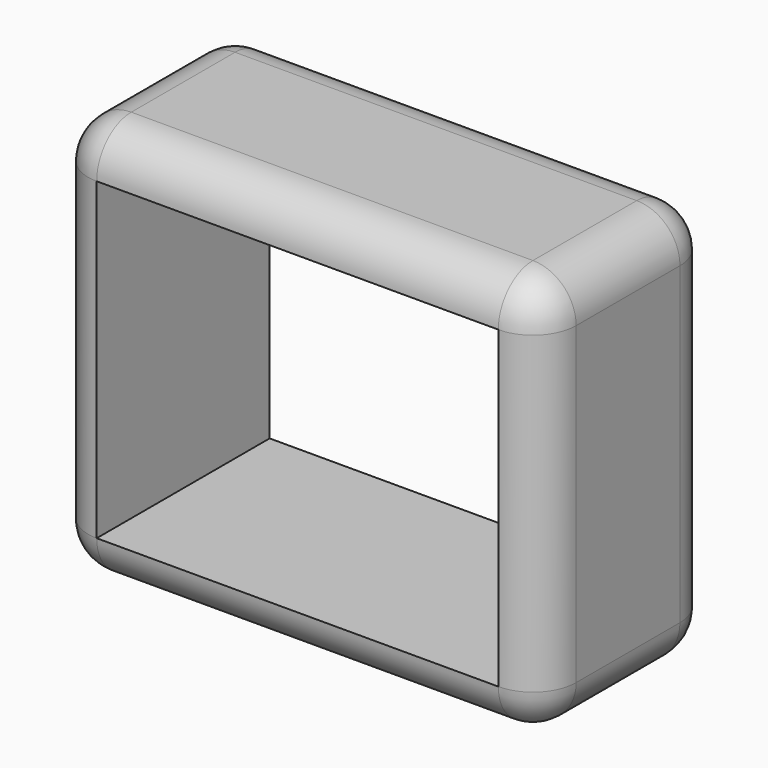
from build123d import *

# Parameters (mm, degrees)
F0_W         = 57.346759364
F0_H         = 47.0794383436
F1_DEPTH     = 25.4
F2_R         = 5.08
F3_T1_DEPTH  = 33.02
F3_T3_DEPTH  = 72.4794383436
F3_S7_W      = 5.08
F3_S7_H      = 5.08
F3_T8_DEPTH  = 5.08
F3_S13_W     = 5.08
F3_S13_H     = 5.08
F3_T14_DEPTH = 5.08
F4_T1_DEPTH  = 47.186759364
F4_T3_DEPTH  = 15.24
F4_T5_DEPTH  = 54.6994383436
F4_S9_W      = 5.08
F4_S9_H      = 5.08
F4_T10_DEPTH = 5.08
F4_S15_W     = 5.08
F4_S15_H     = 5.08
F4_T16_DEPTH = 5.08
F4_S21_W     = 5.08
F4_S21_H     = 5.08
F4_T22_DEPTH = 5.08
F5_T1_DEPTH  = 47.186759364
F5_T3_DEPTH  = 15.24
F5_S7_W      = 5.08
F5_S7_H      = 5.08
F5_T8_DEPTH  = 5.08
F5_S13_W     = 5.08
F5_S13_H     = 5.08
F5_T14_DEPTH = 5.08
F5_T18_ANGLE = 89.9999999979
F6_DEPTH     = 25.4


# Not quite as in the source:
# - a fillet or chamfer that OpenCascade refuses, or shapes differently, is made with other operations: its cross-section is extruded or revolved along the edge and cut away or added


with BuildPart() as f1:
    # F0 (on Front) → F1 (new body)
    with BuildSketch(Plane.XZ):
        with Locations((-1.5025353059, 0.5008457229)):
            Rectangle(F0_W, F0_H)
    extrude(amount=F1_DEPTH)

    # F2
    f2_edges = [f1.edges().sort_by_distance(p)[0] for p in [
        (-30.175915, -25.4, 0.500846),
        (-1.502535, -25.4, -23.038873),
        (27.170844, -25.4, 0.500846),
        (-1.502535, -25.4, 24.040565),
    ]]
    fillet(f2_edges, radius=F2_R)

    # F3: fillet of radius 5.08 on 3 edges, made by hand

    # F3_s2 → F3_t1 (cut)
    with BuildSketch(Plane.XZ.offset(-12.7)):
        with BuildLine():
            ThreePointArc((22.0908443761, 24.0405648947), (25.6829468245, 22.5526673431), (27.1708443761, 18.9605648947))
            Line((27.1708443761, 18.9605648947), (27.1708443761, 24.0405648947))
            Line((27.1708443761, 24.0405648947), (22.0908443761, 24.0405648947))
        make_face()
        with BuildLine():
            ThreePointArc((22.0908443761, -23.038873449), (25.6829468245, -21.5509758974), (27.1708443761, -17.958873449))
            Line((27.1708443761, -17.958873449), (27.1708443761, -23.038873449))
            Line((27.1708443761, -23.038873449), (22.0908443761, -23.038873449))
        make_face()
    extrude(amount=F3_T1_DEPTH, mode=Mode.SUBTRACT)

    # F3_s4 → F3_t3 (cut)
    with BuildSketch(Plane.XY.offset(-35.738873449)):
        with BuildLine():
            ThreePointArc((22.0908443761, 0), (25.6829468245, -1.4878975516), (27.1708443761, -5.08))
            Line((27.1708443761, -5.08), (27.1708443761, 0))
            Line((27.1708443761, 0), (22.0908443761, 0))
        make_face()
    extrude(amount=F3_T3_DEPTH, mode=Mode.SUBTRACT)


with BuildPart() as f3_tool6:
    # F3_s7 → F3_t8 (new body)
    with BuildSketch(Plane.XY.offset(-17.958873449)):
        with Locations((24.6308443761, -22.86)):
            Rectangle(F3_S7_W, F3_S7_H)
    extrude(amount=-F3_T8_DEPTH)

    # F3_s9 → F3_t10 (revolve, cut)
    with BuildSketch(Plane(origin=(22.0908443761, -20.32, -17.958873449), x_dir=(-0.7071067812, 0.7071067812, 0), z_dir=(-0.7071067812, -0.7071067812, 0))):
        with BuildLine():
            ThreePointArc((0, -5.08), (5.08, 0), (0, 5.08))
            Line((0, 5.08), (0, -5.08))
        make_face()
    revolve(axis=Axis((22.0908443761, -20.32, -17.958873449), (0, 0, -1)), mode=Mode.SUBTRACT)


with BuildPart() as f1_1:
    add(f1.part)

    # F3_t5: cut F3_tool6
    add(f3_tool6.part, mode=Mode.SUBTRACT)


with BuildPart() as f3_tool12:
    # F3_s13 → F3_t14 (new body)
    with BuildSketch(Plane.XY.offset(18.9605648947)):
        with Locations((24.6308443761, -22.86)):
            Rectangle(F3_S13_W, F3_S13_H)
    extrude(amount=F3_T14_DEPTH)

    # F3_s15 → F3_t16 (revolve, cut)
    with BuildSketch(Plane(origin=(22.0908443761, -20.32, 18.9605648947), x_dir=(-0.7071067812, 0.7071067812, 0), z_dir=(0.7071067812, 0.7071067812, 0))):
        with BuildLine():
            ThreePointArc((0, -5.08), (5.08, 0), (0, 5.08))
            Line((0, 5.08), (0, -5.08))
        make_face()
    revolve(axis=Axis((22.0908443761, -20.32, 18.9605648947), (0, 0, 1)), mode=Mode.SUBTRACT)


with BuildPart() as f1_2:
    add(f1_1.part)

    # F3_t11: cut F3_tool12
    add(f3_tool12.part, mode=Mode.SUBTRACT)

    # F4: fillet of radius 5.08 on 3 edges, made by hand

    # F4_s2 → F4_t1 (cut)
    with BuildSketch(Plane.YZ.offset(-25.0959149879)):
        with BuildLine():
            ThreePointArc((0, -17.958873449), (-1.4878975516, -21.5509758974), (-5.08, -23.038873449))
            Line((-5.08, -23.038873449), (0, -23.038873449))
            Line((0, -23.038873449), (0, -17.958873449))
        make_face()
    extrude(amount=F4_T1_DEPTH, mode=Mode.SUBTRACT)

    # F4_s4 → F4_t3 (cut)
    with BuildSketch(Plane.XZ.offset(5.08)):
        with BuildLine():
            ThreePointArc((-30.1759149879, -17.958873449), (-28.6880174363, -21.5509758974), (-25.0959149879, -23.038873449))
            Line((-25.0959149879, -23.038873449), (-30.1759149879, -23.038873449))
            Line((-30.1759149879, -23.038873449), (-30.1759149879, -17.958873449))
        make_face()
    extrude(amount=F4_T3_DEPTH, mode=Mode.SUBTRACT)

    # F4_s6 → F4_t5 (cut)
    with BuildSketch(Plane.XY.offset(-17.958873449)):
        with BuildLine():
            ThreePointArc((-30.1759149879, -5.08), (-28.6880174363, -1.4878975516), (-25.0959149879, 0))
            Line((-25.0959149879, 0), (-30.1759149879, 0))
            Line((-30.1759149879, 0), (-30.1759149879, -5.08))
        make_face()
    extrude(amount=F4_T5_DEPTH, mode=Mode.SUBTRACT)


with BuildPart() as f4_tool8:
    # F4_s9 → F4_t10 (new body)
    with BuildSketch(Plane.YZ.offset(-25.0959149879)):
        with Locations((-22.86, -20.498873449)):
            Rectangle(F4_S9_W, F4_S9_H)
    extrude(amount=-F4_T10_DEPTH)

    # F4_s11 → F4_t12 (revolve, cut)
    with BuildSketch(Plane(origin=(-25.0959149879, -20.32, -17.958873449), x_dir=(0, 0.7071067812, 0.7071067812), z_dir=(0, -0.7071067812, 0.7071067812))):
        with BuildLine():
            ThreePointArc((0, -5.08), (5.08, 0), (0, 5.08))
            Line((0, 5.08), (0, -5.08))
        make_face()
    revolve(axis=Axis((-25.0959149879, -20.32, -17.958873449), (-1, 0, 0)), mode=Mode.SUBTRACT)


with BuildPart() as f1_3:
    add(f1_2.part)

    # F4_t7: cut F4_tool8
    add(f4_tool8.part, mode=Mode.SUBTRACT)


with BuildPart() as f4_tool14:
    # F4_s15 → F4_t16 (new body)
    with BuildSketch(Plane.XZ.offset(5.08)):
        with Locations((24.6308443761, -20.498873449)):
            Rectangle(F4_S15_W, F4_S15_H)
    extrude(amount=-F4_T16_DEPTH)

    # F4_s17 → F4_t18 (revolve, cut)
    with BuildSketch(Plane(origin=(22.0908443761, -5.08, -17.958873449), x_dir=(-0.7071067812, 0, 0.7071067812), z_dir=(-0.7071067812, 0, -0.7071067812))):
        with BuildLine():
            ThreePointArc((0, -5.08), (5.08, 0), (0, 5.08))
            Line((0, 5.08), (0, -5.08))
        make_face()
    revolve(axis=Axis((22.0908443761, -5.08, -17.958873449), (0, 1, 0)), mode=Mode.SUBTRACT)


with BuildPart() as f1_4:
    add(f1_3.part)

    # F4_t13: cut F4_tool14
    add(f4_tool14.part, mode=Mode.SUBTRACT)


with BuildPart() as f4_tool20:
    # F4_s21 → F4_t22 (new body)
    with BuildSketch(Plane.YZ.offset(-25.0959149879)):
        with Locations((-2.54, -20.498873449)):
            Rectangle(F4_S21_W, F4_S21_H)
    extrude(amount=-F4_T22_DEPTH)

    # F4_s23 → F4_t24 (revolve, cut)
    with BuildSketch(Plane(origin=(-25.0959149879, -5.08, -17.958873449), x_dir=(0, -0.7071067812, 0.7071067812), z_dir=(0, -0.7071067812, -0.7071067812))):
        with BuildLine():
            ThreePointArc((0, -5.08), (5.08, 0), (0, 5.08))
            Line((0, 5.08), (0, -5.08))
        make_face()
    revolve(axis=Axis((-25.0959149879, -5.08, -17.958873449), (-1, 0, 0)), mode=Mode.SUBTRACT)


with BuildPart() as f1_5:
    add(f1_4.part)

    # F4_t19: cut F4_tool20
    add(f4_tool20.part, mode=Mode.SUBTRACT)

    # F5: fillet of radius 5.08 on 2 edges, made by hand

    # F5_s2 → F5_t1 (cut)
    with BuildSketch(Plane.YZ.offset(-25.0959149879)):
        with BuildLine():
            ThreePointArc((-5.08, 24.0405648947), (-1.4878975516, 22.5526673431), (0, 18.9605648947))
            Line((0, 18.9605648947), (0, 24.0405648947))
            Line((0, 24.0405648947), (-5.08, 24.0405648947))
        make_face()
    extrude(amount=F5_T1_DEPTH, mode=Mode.SUBTRACT)

    # F5_s4 → F5_t3 (cut)
    with BuildSketch(Plane.XZ.offset(5.08)):
        with BuildLine():
            ThreePointArc((-30.1759149879, 18.9605648947), (-28.6880174363, 22.5526673431), (-25.0959149879, 24.0405648947))
            Line((-25.0959149879, 24.0405648947), (-30.1759149879, 24.0405648947))
            Line((-30.1759149879, 24.0405648947), (-30.1759149879, 18.9605648947))
        make_face()
    extrude(amount=F5_T3_DEPTH, mode=Mode.SUBTRACT)


with BuildPart() as f5_tool6:
    # F5_s7 → F5_t8 (new body)
    with BuildSketch(Plane.YZ.offset(-25.0959149879)):
        with Locations((-22.86, 21.5005648947)):
            Rectangle(F5_S7_W, F5_S7_H)
    extrude(amount=-F5_T8_DEPTH)

    # F5_s9 → F5_t10 (revolve, cut)
    with BuildSketch(Plane(origin=(-25.0959149879, -20.32, 18.9605648947), x_dir=(0, 0.7071067812, -0.7071067812), z_dir=(0, 0.7071067812, 0.7071067812))):
        with BuildLine():
            ThreePointArc((0, -5.08), (5.08, 0), (0, 5.08))
            Line((0, 5.08), (0, -5.08))
        make_face()
    revolve(axis=Axis((-25.0959149879, -20.32, 18.9605648947), (-1, 0, 0)), mode=Mode.SUBTRACT)


with BuildPart() as f1_6:
    add(f1_5.part)

    # F5_t5: cut F5_tool6
    add(f5_tool6.part, mode=Mode.SUBTRACT)


with BuildPart() as f5_tool12:
    # F5_s13 → F5_t14 (new body)
    with BuildSketch(Plane.XY.offset(18.9605648947)):
        with Locations((24.6308443761, -2.54)):
            Rectangle(F5_S13_W, F5_S13_H)
    extrude(amount=F5_T14_DEPTH)

    # F5_s15 → F5_t16 (revolve, cut)
    with BuildSketch(Plane(origin=(22.0908443761, -5.08, 18.9605648947), x_dir=(-0.7071067812, -0.7071067812, 0), z_dir=(-0.7071067812, 0.7071067812, 0))):
        with BuildLine():
            ThreePointArc((0, -5.08), (5.08, 0), (0, 5.08))
            Line((0, 5.08), (0, -5.08))
        make_face()
    revolve(axis=Axis((22.0908443761, -5.08, 18.9605648947), (0, 0, 1)), mode=Mode.SUBTRACT)


with BuildPart() as f1_7:
    add(f1_6.part)

    # F5_t11: cut F5_tool12
    add(f5_tool12.part, mode=Mode.SUBTRACT)

    # F5_s17 → F5_t18 (revolve, cut)
    with BuildSketch(Plane.XZ.offset(5.0800000001)):
        with BuildLine():
            ThreePointArc((-30.1759149879, 18.9605648947), (-28.6880174363, 22.5526673431), (-25.0959149879, 24.0405648947))
            Line((-25.0959149879, 24.0405648947), (-30.1759149879, 24.0405648947))
            Line((-30.1759149879, 24.0405648947), (-30.1759149879, 18.9605648947))
        make_face()
    revolve(axis=Axis((-25.0959149878, -5.0800000001, 24.0405648947), (0, 0, -1)), revolution_arc=F5_T18_ANGLE, mode=Mode.SUBTRACT)

    # F6 (cut): a face of the model
    f6_faces = [f1_7.faces().sort_by_distance(p)[0] for p in [
        (-1.5025353059, -25.4, 0.5008457229),
    ]]
    extrude(f6_faces, amount=-F6_DEPTH, mode=Mode.SUBTRACT)


solid = f1_7.part
